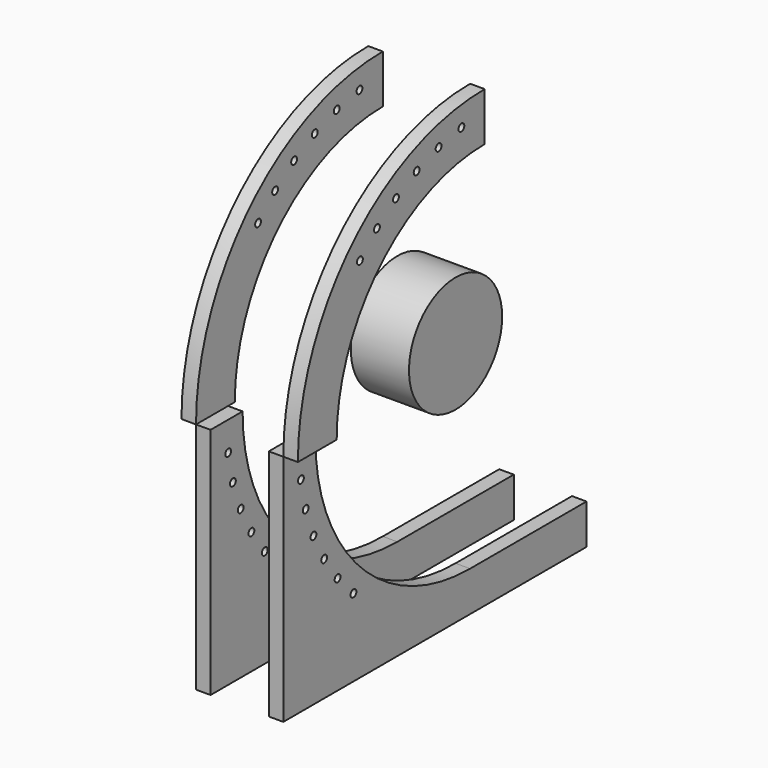
from build123d import *

# Parameters (mm, degrees)
F4_R      = 50.8
F5_DEPTH  = 50.8
F4_R_2    = 3.175
F4_W      = 127
F4_H      = 34.925
F6_DEPTH  = 12.7
F7_DEPTH  = 12.7
F9_R      = 3.175
F10_DEPTH = 12.7


# Not quite as in the source:
# - a variable given as a bare number and used for a length is read in inches; the dataset says mm whatever the document's units were


with BuildPart() as f5:
    # F4 (on offset) → F5 (new body)
    with BuildSketch(Plane.YZ.offset(25.4)):
        with Locations((0, 203.765658)):
            Circle(F4_R)
    extrude(amount=F5_DEPTH)


with BuildPart() as f6:
    # F4 (on offset) → F6 (new body)
    with BuildSketch(Plane.YZ.offset(25.4)):
        with BuildLine():
            ThreePointArc((-203.765658, 203.765658), (-144.0840785447, 59.6815794553), (0, 0))
            Line((0, 0), (0, 34.925))
            ThreePointArc((0, 34.925), (-119.3883742118, 84.3772837882), (-168.840658, 203.765658))
            Line((-168.840658, 203.765658), (-203.765658, 203.765658))
        make_face()
        with Locations((-127.2828635618, 67.7217705068)):
            Circle(F4_R_2, mode=Mode.SUBTRACT)
        with Locations((-144.6045721292, 86.2991334064)):
            Circle(F4_R_2, mode=Mode.SUBTRACT)
        with Locations((-159.2384059639, 107.0599355899)):
            Circle(F4_R_2, mode=Mode.SUBTRACT)
        with Locations((-170.9123549098, 129.6182802988)):
            Circle(F4_R_2, mode=Mode.SUBTRACT)
        with Locations((-179.409426434, 153.5548584902)):
            Circle(F4_R_2, mode=Mode.SUBTRACT)
        with Locations((-184.5716790307, 178.4247428512)):
            Circle(F4_R_2, mode=Mode.SUBTRACT)
        with Locations((63.5, 17.4625)):
            Rectangle(F4_W, F4_H)
    extrude(amount=F6_DEPTH)

    # F4 (on offset) → F7 (join)
    with BuildSketch(Plane.YZ.offset(25.4)):
        with BuildLine():
            Line((-203.765658, 0), (0, 0))
            ThreePointArc((0, 0), (-144.0840785447, 59.6815794553), (-203.765658, 203.765658))
            Line((-203.765658, 203.765658), (-203.765658, 0))
        make_face()
    extrude(amount=F7_DEPTH)


with BuildPart() as f10:
    # F9 (on offset) → F10 (new body)
    with BuildSketch(Plane.YZ.offset(38.1)):
        with BuildLine():
            ThreePointArc((-161.449258, 203.765658), (-114.1618651493, 317.9275231493), (0, 365.214916))
            Line((0, 365.214916), (0, 407.531316))
            ThreePointArc((0, 407.531316), (-144.0840785447, 347.8497365447), (-203.765658, 203.765658))
            Line((-203.765658, 203.765658), (-161.449258, 203.765658))
        make_face()
        with Locations((-136.0846270462, 331.0049638865)):
            Circle(F9_R, mode=Mode.SUBTRACT)
        with Locations((-117.5128102236, 348.3326186588)):
            Circle(F9_R, mode=Mode.SUBTRACT)
        with Locations((-96.7566937712, 362.9730978112)):
            Circle(F9_R, mode=Mode.SUBTRACT)
        with Locations((-74.20208735, 374.6542676663)):
            Circle(F9_R, mode=Mode.SUBTRACT)
        with Locations((-50.2682305166, 383.1590014704)):
            Circle(F9_R, mode=Mode.SUBTRACT)
        with Locations((-25.4, 388.3292152933)):
            Circle(F9_R, mode=Mode.SUBTRACT)
    extrude(amount=F10_DEPTH)


with BuildPart() as f11_1:
    # F11: instance of F10
    add(f10.part.mirror(Plane.YZ))


with BuildPart() as f11_2:
    # F11: instance of F5
    add(f5.part.mirror(Plane.YZ))


with BuildPart() as f11_3:
    # F11: instance of F6
    add(f6.part.mirror(Plane.YZ))


with BuildPart() as f5_1:
    # F13: moved
    add(f5.part.moved(Location((-50.8, 0, 0))))


solid = Compound([f6.part, f10.part, f11_1.part, f11_3.part, f5_1.part])
